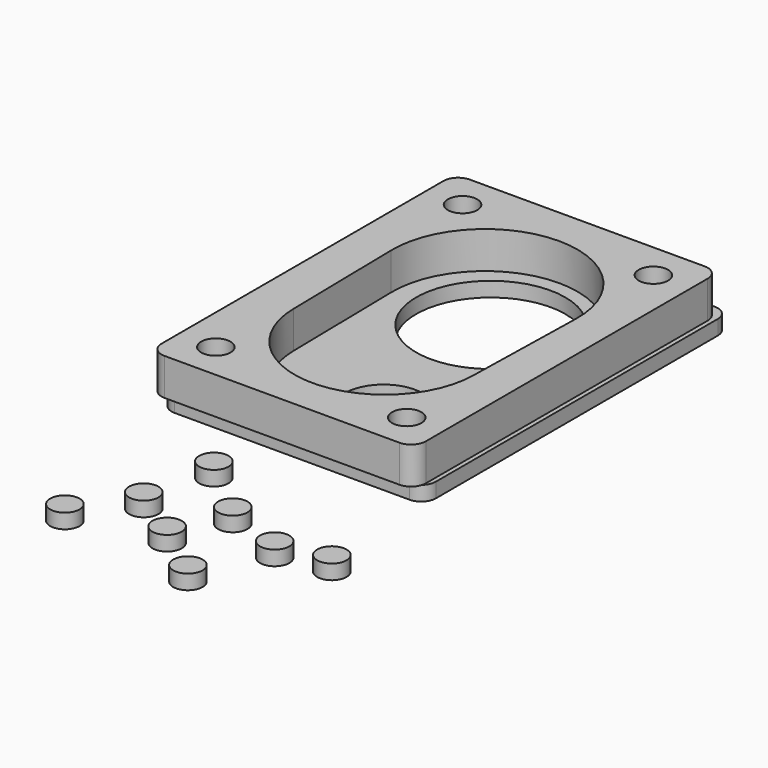
from build123d import *

# Parameters (mm, degrees)
F0_R     = 6.35
F2_DEPTH = 3.175
F0_R_2   = 16.891
F0_R_3   = 32.258
F3_DEPTH = 6.35
F1_R     = 6.35
F4_DEPTH = 5.842
F5_DEPTH = 16.002
F6_R     = 6.35
F7_DEPTH = 6.35


with BuildPart() as f2:
    # F0 (on Top) → F2 (new body)
    with BuildSketch(Plane.XY):
        with Locations((-41.275, -66.675)):
            Circle(F0_R)
    extrude(amount=-F2_DEPTH)



with BuildPart() as f2b:
    # F0 (on Top) → F2, piece 2 (new body)
    with BuildSketch(Plane.XY):
        with Locations((-41.275, 66.675)):
            Circle(F0_R)
    extrude(amount=-F2_DEPTH)


with BuildPart() as f2c:
    # F0 (on Top) → F2, piece 3 (new body)
    with BuildSketch(Plane.XY):
        with Locations((41.275, 66.675)):
            Circle(F0_R)
    extrude(amount=-F2_DEPTH)


with BuildPart() as f2d:
    # F0 (on Top) → F2, piece 4 (new body)
    with BuildSketch(Plane.XY):
        with Locations((41.275, -66.675)):
            Circle(F0_R)
    extrude(amount=-F2_DEPTH)


with BuildPart() as f2_1:
    add(f2.part)

    add(f2b.part)  # F3 merges F2b

    add(f2c.part)  # F3 merges F2c

    add(f2d.part)  # F3 merges F2d
    # F0 (on Top) → F3 (join)
    with BuildSketch(Plane.XY):
        with BuildLine():
            Line((-50.8, -82.55), (50.8, -82.55))
            ThreePointArc((50.8, -82.55), (55.2901280605, -80.6901280605), (57.15, -76.2))
            Line((57.15, -76.2), (57.15, 76.2))
            ThreePointArc((57.15, 76.2), (55.2901280605, 80.6901280605), (50.8, 82.55))
            Line((50.8, 82.55), (-50.8, 82.55))
            ThreePointArc((-50.8, 82.55), (-55.2901280605, 80.6901280605), (-57.15, 76.2))
            Line((-57.15, 76.2), (-57.15, -76.2))
            ThreePointArc((-57.15, -76.2), (-55.2901280605, -80.6901280605), (-50.8, -82.55))
        make_face()
        with Locations((-41.275, -66.675)):
            Circle(F0_R, mode=Mode.SUBTRACT)
        with Locations((9.525, -44.958)):
            Circle(F0_R_2, mode=Mode.SUBTRACT)
        with Locations((41.275, -66.675)):
            Circle(F0_R, mode=Mode.SUBTRACT)
        with Locations((-41.275, 66.675)):
            Circle(F0_R, mode=Mode.SUBTRACT)
        with Locations((0, 24.892)):
            Circle(F0_R_3, mode=Mode.SUBTRACT)
        with Locations((41.275, 66.675)):
            Circle(F0_R, mode=Mode.SUBTRACT)
    extrude(amount=-F3_DEPTH)


with BuildPart() as f4:
    # F1 (on Top) → F4 (new body)
    with BuildSketch(Plane.XY):
        with Locations((39.384733719, 63.5895566996)):
            Circle(F1_R)
    extrude(amount=F4_DEPTH)



with BuildPart() as f4b:
    # F1 (on Top) → F4, piece 2 (new body)
    with BuildSketch(Plane.XY):
        with Locations((-43.165266281, 63.5895566996)):
            Circle(F1_R)
    extrude(amount=F4_DEPTH)


with BuildPart() as f4c:
    # F1 (on Top) → F4, piece 3 (new body)
    with BuildSketch(Plane.XY):
        with Locations((-43.165266281, -69.7604433004)):
            Circle(F1_R)
    extrude(amount=F4_DEPTH)


with BuildPart() as f4d:
    # F1 (on Top) → F4, piece 4 (new body)
    with BuildSketch(Plane.XY):
        with Locations((39.384733719, -69.7604433004)):
            Circle(F1_R)
    extrude(amount=F4_DEPTH)


with BuildPart() as f4_1:
    add(f4.part)

    add(f4b.part)  # F5 merges F4b

    add(f4c.part)  # F5 merges F4c

    add(f4d.part)  # F5 merges F4d
    # F1 (on Top) → F5 (join)
    with BuildSketch(Plane.XY):
        with BuildLine():
            Line((-52.690266281, -85.6354433004), (48.909733719, -85.6354433004))
            ThreePointArc((48.909733719, -85.6354433004), (53.3998617796, -83.7755713609), (55.259733719, -79.2854433004))
            Line((55.259733719, -79.2854433004), (55.259733719, 73.1145566996))
            ThreePointArc((55.259733719, 73.1145566996), (53.3998617796, 77.6046847601), (48.909733719, 79.4645566996))
            Line((48.909733719, 79.4645566996), (-52.690266281, 79.4645566996))
            ThreePointArc((-52.690266281, 79.4645566996), (-57.1803943415, 77.6046847601), (-59.040266281, 73.1145566996))
            Line((-59.040266281, 73.1145566996), (-59.040266281, -79.2854433004))
            ThreePointArc((-59.040266281, -79.2854433004), (-57.1803943415, -83.7755713609), (-52.690266281, -85.6354433004))
        make_face()
        with Locations((-43.165266281, -69.7604433004)):
            Circle(F1_R, mode=Mode.SUBTRACT)
        with Locations((39.384733719, -69.7604433004)):
            Circle(F1_R, mode=Mode.SUBTRACT)
        with BuildLine():
            ThreePointArc((-41.1198244616, 22.3061300117), (-1.1151278345, 63.2139243167), (38.8841910485, 22.3008716804))
            Line((38.8841910485, 22.3008716804), (37.668826681, -31.6604433004))
            ThreePointArc((37.668826681, -31.6604433004), (-1.2486367631, -69.896214704), (-40.1661002073, -31.6604433004))
            Line((-40.1661002073, -31.6604433004), (-41.1198244616, 22.3061300117))
        make_face(mode=Mode.SUBTRACT)
        with Locations((-43.165266281, 63.5895566996)):
            Circle(F1_R, mode=Mode.SUBTRACT)
        with Locations((39.384733719, 63.5895566996)):
            Circle(F1_R, mode=Mode.SUBTRACT)
    extrude(amount=F5_DEPTH)


with BuildPart() as f7:
    # F6 (on Top) → F7 (new body)
    with BuildSketch(Plane.XY):
        with Locations((29.8007111996, -176.0796308517)):
            Circle(F6_R)
    extrude(amount=-F7_DEPTH)


with BuildPart() as f7b:
    # F6 (on Top) → F7, piece 2 (new body)
    with BuildSketch(Plane.XY):
        with Locations((63.177511096, -139.9782001972)):
            Circle(F6_R)
    extrude(amount=-F7_DEPTH)


with BuildPart() as f7c:
    # F6 (on Top) → F7, piece 3 (new body)
    with BuildSketch(Plane.XY):
        with Locations((41.7209938169, -144.065156579)):
            Circle(F6_R)
    extrude(amount=-F7_DEPTH)


with BuildPart() as f7d:
    # F6 (on Top) → F7, piece 4 (new body)
    with BuildSketch(Plane.XY):
        with Locations((6.6412999295, -158.3694964647)):
            Circle(F6_R)
    extrude(amount=-F7_DEPTH)


with BuildPart() as f7e:
    # F6 (on Top) → F7, piece 5 (new body)
    with BuildSketch(Plane.XY):
        with Locations((-30.4818730801, -167.2245711088)):
            Circle(F6_R)
    extrude(amount=-F7_DEPTH)


with BuildPart() as f7f:
    # F6 (on Top) → F7, piece 6 (new body)
    with BuildSketch(Plane.XY):
        with Locations((-15.1557931677, -143.7245756388)):
            Circle(F6_R)
    extrude(amount=-F7_DEPTH)


with BuildPart() as f7g:
    # F6 (on Top) → F7, piece 7 (new body)
    with BuildSketch(Plane.XY):
        with Locations((15.1557894424, -133.5071921349)):
            Circle(F6_R)
    extrude(amount=-F7_DEPTH)


with BuildPart() as f7h:
    # F6 (on Top) → F7, piece 8 (new body)
    with BuildSketch(Plane.XY):
        with Locations((-10.7282577083, -111.3695204258)):
            Circle(F6_R)
    extrude(amount=-F7_DEPTH)


solid = Compound([f2_1.part, f4_1.part, f7.part, f7b.part, f7c.part, f7d.part, f7e.part, f7f.part, f7g.part, f7h.part])
